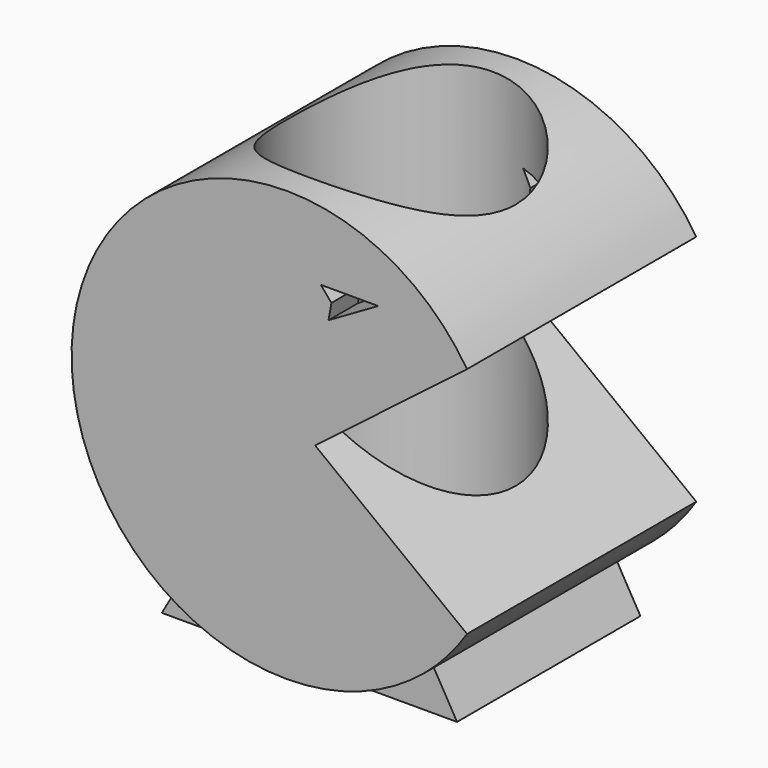
from build123d import *

# Parameters (mm, degrees)
F1_DEPTH      = 25
F2_DEPTH      = 20
F3_R          = 20
F4_DEPTH      = 30
F4_DEPTH_BACK = 37.501
F5_TEXT_SIZE  = 4.9992188721
F6_DEPTH      = 0.5


# Not quite as in the source:
# - Text() gives the source's letters only with a copy of the font that has no kerning and outlines rounded to 1/6400 em; it was checked with that copy


with BuildPart() as f1:
    # F0 (on Front) → F1 (new body, symmetric)
    with BuildSketch(Plane.XZ):
        with BuildLine():
            Line((5, 0), (31.5055376321, 20.338414356))
            ThreePointArc((31.5055376321, 20.338414356), (-25.953035772, 27.0682458651), (-21.6451688735, -30.622486255))
            ThreePointArc((-21.6451688735, -30.622486255), (0, -37.5), (21.6451688735, -30.622486255))
            ThreePointArc((21.6451688735, -30.622486255), (27.0682458651, -25.953035772), (31.5055376321, -20.338414356))
            Line((31.5055376321, -20.338414356), (5, 0))
        make_face()
        Polygon((6, 25), (16, 25), (7.3397459622, 20), (7.8356421265, 22.8123669011), align=None, mode=Mode.SUBTRACT)
    extrude(amount=F1_DEPTH, both=True)

    # F0 (on Front) → F2 (join, symmetric)
    with BuildSketch(Plane.XZ):
        with BuildLine():
            ThreePointArc((21.6451688735, -30.622486255), (0, -37.5), (-21.6451688735, -30.622486255))
            Line((-21.6451688735, -30.622486255), (-25.7602408528, -37.75))
            Line((-25.7602408528, -37.75), (25.7602408528, -37.75))
            Line((25.7602408528, -37.75), (21.6451688735, -30.622486255))
        make_face()
    extrude(amount=F2_DEPTH, both=True)

    # F3 (on Top) → F4 (cut, two sides)
    with BuildSketch(Plane.XY) as f4_sk:
        Circle(F3_R)
    extrude(amount=-F4_DEPTH, mode=Mode.SUBTRACT)
    extrude(f4_sk.sketch, amount=F4_DEPTH_BACK, mode=Mode.SUBTRACT)

    # F5 (on face) → F6 (cut)
    with BuildSketch(Plane(origin=(0, 0, -37.75), x_dir=(1, 0, 0), z_dir=(0, 0, -1))):
        with Locations((-15, 8.4005624121)):
            Text('CREATED BY:', F5_TEXT_SIZE, font='Open Sans', text_align=(TextAlign.LEFT, TextAlign.BOTTOM))
        with Locations((-15, 1.6016247461)):
            Text('AJ JOHNSON', F5_TEXT_SIZE, font='Open Sans', text_align=(TextAlign.LEFT, TextAlign.BOTTOM))
        with Locations((-13.7009842212, -5.1973129199)):
            Text('1ST GRADE', F5_TEXT_SIZE, font='Open Sans', text_align=(TextAlign.LEFT, TextAlign.BOTTOM))
        with Locations((-8.5049211061, -11.9962505858)):
            Text('2017', F5_TEXT_SIZE, font='Open Sans', text_align=(TextAlign.LEFT, TextAlign.BOTTOM))
    extrude(amount=-F6_DEPTH, mode=Mode.SUBTRACT)


solid = f1.part
